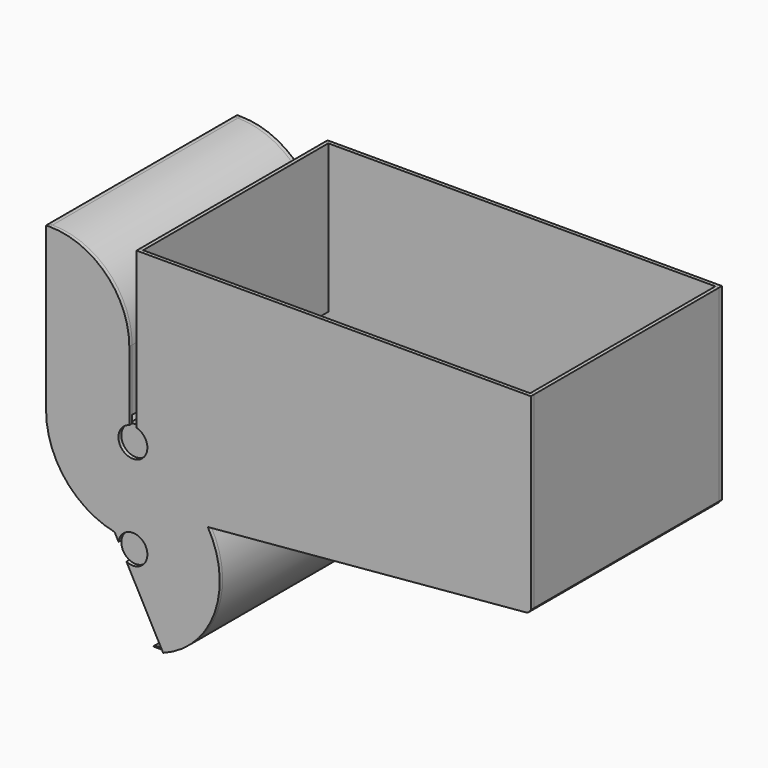
from build123d import *

# Parameters (mm, degrees)
F0_R     = 25.4
F1_DEPTH = 406.4
F0_W     = 6.35
F0_H     = 260.35
F3_DEPTH = 6.35
F5_DEPTH = 6.35


# Not quite as in the source:
# - a feature names something its author has since deleted; it is built from what else it names


with BuildPart() as f1:
    # F0 (on Front) → F1 (new body)
    with BuildSketch(Plane.XZ):
        with Locations((0, 146.05)):
            Circle(F0_R)
    extrude(amount=F1_DEPTH)


with BuildPart() as f1b:
    # F0 (on Front) → F1, piece 2 (new body)
    with BuildSketch(Plane.XZ):
        with BuildLine():
            Line((-32.1996567388, 162.1904682274), (-30.8580043747, 168.3971153846))
            ThreePointArc((-30.8580043747, 168.3971153846), (-113.6604901426, 219.4336138929), (-146.05, 311.15))
            Line((-146.05, 311.15), (-146.05, 457.2))
            Line((-146.05, 457.2), (-152.4, 457.2))
            Line((-152.4, 457.2), (-152.4, 311.15))
            ThreePointArc((-152.4, 311.15), (-118.6022505836, 215.4459449318), (-32.1996567388, 162.1904682274))
        make_face()
    extrude(amount=F1_DEPTH)


with BuildPart() as f1c:
    # F0 (on Front) → F1, piece 3 (new body)
    with BuildSketch(Plane.XZ):
        with Locations((0, 311.15)):
            Circle(F0_R)
    extrude(amount=F1_DEPTH)


with BuildPart() as f1d:
    # F0 (on Front) → F1, piece 4 (new body)
    with BuildSketch(Plane.XZ):
        with BuildLine():
            ThreePointArc((120.4827788524, 228.6), (135.5987911183, 91.7953195822), (30.287569645, 3.175))
            Line((30.287569645, 3.175), (53.032955556, 3.175))
            ThreePointArc((53.032955556, 3.175), (143.559051356, 94.8976904357), (131.430489055, 223.1978226963))
            Line((131.430489055, 223.1978226963), (692.7120644971, 273.0749242296))
            Line((692.7120644971, 273.0749242296), (698.5, 279.4))
            Line((698.5, 279.4), (698.5, 609.6))
            Line((698.5, 609.6), (692.15, 609.6))
            Line((692.15, 609.6), (692.15, 279.4))
            Line((692.15, 279.4), (120.4827788524, 228.6))
        make_face()
    extrude(amount=F1_DEPTH)


with BuildPart() as f1e:
    # F0 (on Front) → F1, piece 5 (new body)
    with BuildSketch(Plane.XZ):
        with Locations((9.525, 479.425)):
            Rectangle(F0_W, F0_H)
    extrude(amount=F1_DEPTH)


with BuildPart() as f1f:
    # F0 (on Front) → F1, piece 6 (new body)
    with BuildSketch(Plane.XZ):
        with BuildLine():
            Line((-12.7, 457.2), (-12.7, 349.25))
            Line((-12.7, 349.25), (-6.35, 349.25))
            Line((-6.35, 349.25), (-6.35, 457.2))
            ThreePointArc((-6.35, 457.2), (-47.2671826682, 555.9828173318), (-146.05, 596.9))
            Line((-146.05, 596.9), (-152.4, 596.9))
            Line((-152.4, 596.9), (-152.4, 590.55))
            Line((-152.4, 590.55), (-146.05, 590.55))
            ThreePointArc((-146.05, 590.55), (-51.7573107288, 551.4926892712), (-12.7, 457.2))
        make_face()
    extrude(amount=F1_DEPTH)


with BuildPart() as f3:
    # F2 (on Front) → F3 (new body)
    with BuildSketch(Plane.XZ):
        with BuildLine():
            Line((692.7120644971, 273.0749242296), (698.5, 279.4))
            Line((698.5, 279.4), (698.5, 609.6))
            Line((698.5, 609.6), (692.15, 609.6))
            Line((692.15, 609.6), (6.35, 609.6))
            Line((6.35, 609.6), (6.35, 349.25))
            Line((6.35, 349.25), (-6.35, 349.25))
            Line((-6.35, 349.25), (-6.35, 457.2))
            ThreePointArc((-6.35, 457.2), (-47.2671826682, 555.9828173318), (-146.05, 596.9))
            Line((-146.05, 596.9), (-152.4, 596.9))
            Line((-152.4, 596.9), (-152.4, 457.2))
            Line((-152.4, 457.2), (-152.4, 311.15))
            ThreePointArc((-152.4, 311.15), (-118.6022505836, 215.4459449318), (-32.1996567388, 162.1904682274))
            Line((-32.1996567388, 162.1904682274), (53.032955556, 3.175))
            ThreePointArc((53.032955556, 3.175), (143.559051356, 94.8976904357), (131.430489055, 223.1978226963))
            Line((131.430489055, 223.1978226963), (692.7120644971, 273.0749242296))
        make_face()
    extrude(amount=-F3_DEPTH)


with BuildPart() as f5:
    # F4 (on face) → F5 (new body)
    with BuildSketch(Plane.XZ.offset(406.4)):
        with BuildLine():
            Line((-6.35, 349.25), (-6.35, 457.2))
            ThreePointArc((-6.35, 457.2), (-47.2671826682, 555.9828173318), (-146.05, 596.9))
            Line((-146.05, 596.9), (-152.4, 596.9))
            Line((-152.4, 596.9), (-152.4, 457.2))
            Line((-152.4, 457.2), (-152.4, 311.15))
            ThreePointArc((-152.4, 311.15), (-118.6022505836, 215.4459449318), (-32.1996567388, 162.1904682274))
            Line((-32.1996567388, 162.1904682274), (-25.2100838748, 149.1502695083))
            ThreePointArc((-25.2100838748, 149.1502695083), (1.5530404984, 171.4024765104), (25.4, 146.05))
            ThreePointArc((25.4, 146.05), (13.3457878073, 124.4386615916), (-11.3755864411, 123.3397372732))
            Line((-11.3755864411, 123.3397372732), (53.032955556, 3.175))
            ThreePointArc((53.032955556, 3.175), (143.559051356, 94.8976904357), (131.430489055, 223.1978226963))
            Line((131.430489055, 223.1978226963), (692.7120644971, 273.0749242296))
            Line((692.7120644971, 273.0749242296), (698.5, 279.4))
            Line((698.5, 279.4), (698.5, 609.6))
            Line((698.5, 609.6), (6.35, 609.6))
            Line((6.35, 609.6), (6.35, 349.25))
            Line((6.35, 349.25), (6.35, 335.7434442484))
            ThreePointArc((6.35, 335.7434442484), (0, 285.75), (-6.35, 335.7434442484))
            Line((-6.35, 335.7434442484), (-6.35, 349.25))
        make_face()
    extrude(amount=F5_DEPTH)


solid = Compound([f1.part, f1b.part, f1c.part, f1d.part, f1e.part, f1f.part, f3.part, f5.part])
